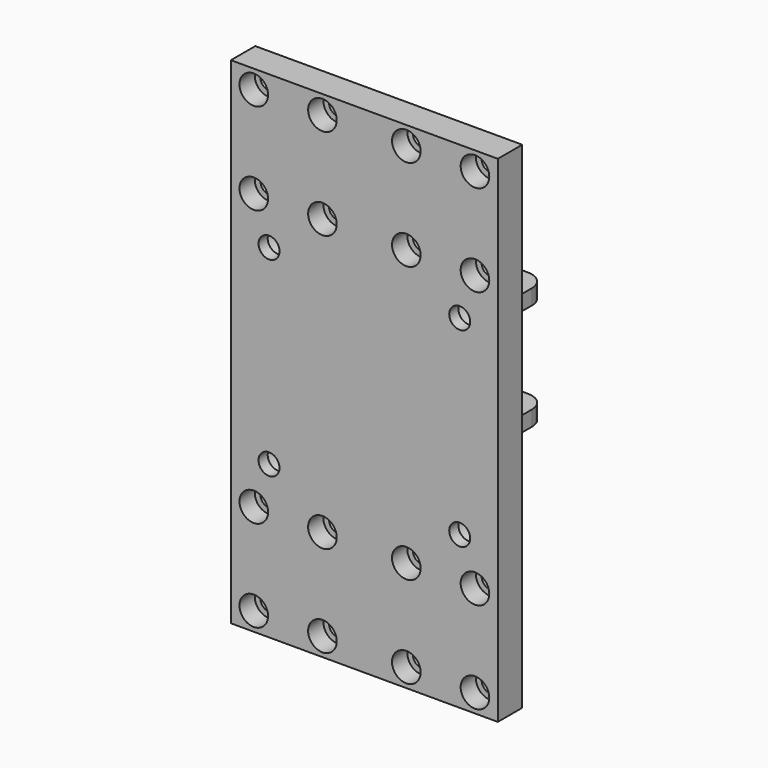
from build123d import *

# Parameters (mm, degrees)
F0_W      = 70
F0_H      = 130
F0_R      = 2.25
F1_DEPTH  = 8
F3_W      = 13
F3_H      = 24
F4_DEPTH  = 30
F5_R      = 1.8965654334
F5_R_2    = 5.25
F6_DEPTH  = 41.501
F7_R      = 2.75
F8_DEPTH  = 8.001
F9_R      = 5
F9_R_2    = 2.75
F10_DEPTH = 5
F11_W     = 13
F11_H     = 30
F12_DEPTH = 4
F13_W     = 13
F13_H     = 30
F14_DEPTH = 4
F15_R     = 3.75
F15_R_2   = 2.25
F16_DEPTH = 5
F17_DEPTH = 4
F18_DEPTH = 4


# Not quite as in the source:
# - a feature names something its author has since deleted; it is built from what else it names


with BuildPart() as f1:
    # F0 (on Front) → F1 (new body)
    with BuildSketch(Plane.XZ):
        with Locations((35, 65)):
            Rectangle(F0_W, F0_H)
        with Locations((6, 4.8520950079)):
            Circle(F0_R, mode=Mode.SUBTRACT)
        with Locations((6, 28.8520950079)):
            Circle(F0_R, mode=Mode.SUBTRACT)
        with Locations((24, 4.8520950079)):
            Circle(F0_R, mode=Mode.SUBTRACT)
        with Locations((24, 28.8520950079)):
            Circle(F0_R, mode=Mode.SUBTRACT)
        with Locations((46, 4.8520950079)):
            Circle(F0_R, mode=Mode.SUBTRACT)
        with Locations((46, 28.8520950079)):
            Circle(F0_R, mode=Mode.SUBTRACT)
        with Locations((64, 4.8520950079)):
            Circle(F0_R, mode=Mode.SUBTRACT)
        with Locations((64, 28.8520950079)):
            Circle(F0_R, mode=Mode.SUBTRACT)
        with Locations((6, 101.1479049921)):
            Circle(F0_R, mode=Mode.SUBTRACT)
        with Locations((6, 125.1479049921)):
            Circle(F0_R, mode=Mode.SUBTRACT)
        with Locations((24, 101.1479049921)):
            Circle(F0_R, mode=Mode.SUBTRACT)
        with Locations((24, 125.1479049921)):
            Circle(F0_R, mode=Mode.SUBTRACT)
        with Locations((46, 101.1479049921)):
            Circle(F0_R, mode=Mode.SUBTRACT)
        with Locations((46, 125.1479049921)):
            Circle(F0_R, mode=Mode.SUBTRACT)
        with Locations((64, 101.1479049921)):
            Circle(F0_R, mode=Mode.SUBTRACT)
        with Locations((64, 125.1479049921)):
            Circle(F0_R, mode=Mode.SUBTRACT)
    extrude(amount=-F1_DEPTH)

    # F3 (on face) → F4 (join)
    with BuildSketch(Plane(origin=(0, 8, 0), x_dir=(-1, 0, 0), z_dir=(0, 1, 0))):
        with Locations((-35, 65)):
            Rectangle(F3_W, F3_H)
    extrude(amount=F4_DEPTH)

    # F5 (on face) → F6 (cut, through all)
    with BuildSketch(Plane(origin=(28.5, 0, 0), x_dir=(0, -1, 0), z_dir=(-1, 0, 0))):
        with Locations((-32, 65)):
            Circle(F5_R)
        with Locations((-24, 73)):
            Circle(F5_R)
        with Locations((-16, 65)):
            Circle(F5_R)
        with Locations((-24, 57)):
            Circle(F5_R)
        with Locations((-24, 65)):
            Circle(F5_R_2)
    extrude(amount=-F6_DEPTH, mode=Mode.SUBTRACT)

    # F7 (on face) → F8 (cut, through all)
    with BuildSketch(Plane(origin=(0, 8, 0), x_dir=(-1, 0, 0), z_dir=(0, 1, 0))):
        with Locations((-60, 90)):
            Circle(F7_R)
        with Locations((-10, 90)):
            Circle(F7_R)
        with Locations((-60, 40)):
            Circle(F7_R)
        with Locations((-10, 40)):
            Circle(F7_R)
    extrude(amount=-F8_DEPTH, mode=Mode.SUBTRACT)

    # F9 (on face) → F10 (cut)
    with BuildSketch(Plane(origin=(0, 8, 0), x_dir=(-1, 0, 0), z_dir=(0, 1, 0))):
        with Locations((-60, 90)):
            Circle(F9_R)
        with Locations((-60, 90)):
            Circle(F9_R_2, mode=Mode.SUBTRACT)
        with Locations((-10, 90)):
            Circle(F9_R)
        with Locations((-10, 90)):
            Circle(F9_R_2, mode=Mode.SUBTRACT)
        with Locations((-10, 40)):
            Circle(F9_R)
        with Locations((-10, 40)):
            Circle(F9_R_2, mode=Mode.SUBTRACT)
        with Locations((-60, 40)):
            Circle(F9_R)
        with Locations((-60, 40)):
            Circle(F9_R_2, mode=Mode.SUBTRACT)
    extrude(amount=-F10_DEPTH, mode=Mode.SUBTRACT)

    # F11 (on face) → F12 (join)
    with BuildSketch(Plane.XY.offset(77)):
        with Locations((35, 23)):
            Rectangle(F11_W, F11_H)
    extrude(amount=F12_DEPTH)

    # F13 (on face) → F14 (join)
    with BuildSketch(Plane(origin=(0, 0, 53), x_dir=(1, 0, 0), z_dir=(0, 0, -1))):
        with Locations((35, -23)):
            Rectangle(F13_W, F13_H)
    extrude(amount=F14_DEPTH)

    # F15 (on face) → F16 (cut)
    with BuildSketch(Plane.XZ):
        with Locations((6, 125.1479049921)):
            Circle(F15_R)
        with Locations((6, 125.1479049921)):
            Circle(F15_R_2, mode=Mode.SUBTRACT)
        with Locations((24, 101.1479049921)):
            Circle(F15_R)
        with Locations((24, 101.1479049921)):
            Circle(F15_R_2, mode=Mode.SUBTRACT)
        with Locations((24, 125.1479049921)):
            Circle(F15_R)
        with Locations((24, 125.1479049921)):
            Circle(F15_R_2, mode=Mode.SUBTRACT)
        with Locations((6, 101.1479049921)):
            Circle(F15_R)
        with Locations((6, 101.1479049921)):
            Circle(F15_R_2, mode=Mode.SUBTRACT)
        with Locations((46, 125.1479049921)):
            Circle(F15_R)
        with Locations((46, 125.1479049921)):
            Circle(F15_R_2, mode=Mode.SUBTRACT)
        with Locations((64, 125.1479049921)):
            Circle(F15_R)
        with Locations((64, 125.1479049921)):
            Circle(F15_R_2, mode=Mode.SUBTRACT)
        with Locations((46, 101.1479049921)):
            Circle(F15_R)
        with Locations((46, 101.1479049921)):
            Circle(F15_R_2, mode=Mode.SUBTRACT)
        with Locations((64, 101.1479049921)):
            Circle(F15_R)
        with Locations((64, 101.1479049921)):
            Circle(F15_R_2, mode=Mode.SUBTRACT)
        with Locations((6, 28.8520950079)):
            Circle(F15_R)
        with Locations((6, 28.8520950079)):
            Circle(F15_R_2, mode=Mode.SUBTRACT)
        with Locations((24, 28.8520950079)):
            Circle(F15_R)
        with Locations((24, 28.8520950079)):
            Circle(F15_R_2, mode=Mode.SUBTRACT)
        with Locations((46, 28.8520950079)):
            Circle(F15_R)
        with Locations((46, 28.8520950079)):
            Circle(F15_R_2, mode=Mode.SUBTRACT)
        with Locations((6, 4.8520950079)):
            Circle(F15_R)
        with Locations((6, 4.8520950079)):
            Circle(F15_R_2, mode=Mode.SUBTRACT)
        with Locations((64, 28.8520950079)):
            Circle(F15_R)
        with Locations((64, 28.8520950079)):
            Circle(F15_R_2, mode=Mode.SUBTRACT)
        with Locations((24, 4.8520950079)):
            Circle(F15_R)
        with Locations((24, 4.8520950079)):
            Circle(F15_R_2, mode=Mode.SUBTRACT)
        with Locations((46, 4.8520950079)):
            Circle(F15_R)
        with Locations((46, 4.8520950079)):
            Circle(F15_R_2, mode=Mode.SUBTRACT)
        with Locations((64, 4.8520950079)):
            Circle(F15_R)
        with Locations((64, 4.8520950079)):
            Circle(F15_R_2, mode=Mode.SUBTRACT)
    extrude(amount=-F16_DEPTH, mode=Mode.SUBTRACT)

    # F13 (on face) → F17 (join)
    with BuildSketch(Plane(origin=(0, 0, 53), x_dir=(1, 0, 0), z_dir=(0, 0, -1))):
        with BuildLine():
            Line((52.5, -8), (52.4993246093, -8))
            Line((52.4993246093, -8), (41.5, -8))
            Line((41.5, -8), (41.5, -38))
            Line((41.5, -38), (47.5, -38))
            ThreePointArc((47.5, -38), (51.0355339059, -36.5355339059), (52.5, -33))
            Line((52.5, -33), (52.5, -8))
        make_face()
        with BuildLine():
            Line((28.5, -38), (28.5, -8))
            Line((28.5, -8), (17.5, -8))
            Line((17.5, -8), (17.5, -33))
            ThreePointArc((17.5, -33), (18.9644660941, -36.5355339059), (22.5, -38))
            Line((22.5, -38), (28.5, -38))
        make_face()
    extrude(amount=F17_DEPTH)

    # F11 (on face) → F18 (join)
    with BuildSketch(Plane.XY.offset(77)):
        with BuildLine():
            Line((28.5, 8), (28.5, 38))
            Line((28.5, 38), (22.5, 38))
            ThreePointArc((22.5, 38), (18.9644660941, 36.5355339059), (17.5, 33))
            Line((17.5, 33), (17.5, 8))
            Line((17.5, 8), (28.5, 8))
        make_face()
        with BuildLine():
            Line((47.5, 38), (41.5, 38))
            Line((41.5, 38), (41.5, 8))
            Line((41.5, 8), (52.5, 8))
            Line((52.5, 8), (52.5, 33))
            ThreePointArc((52.5, 33), (51.0355339059, 36.5355339059), (47.5, 38))
        make_face()
        with Locations((35, 23)):
            Rectangle(F11_W, F11_H)
    extrude(amount=F18_DEPTH)


solid = f1.part
